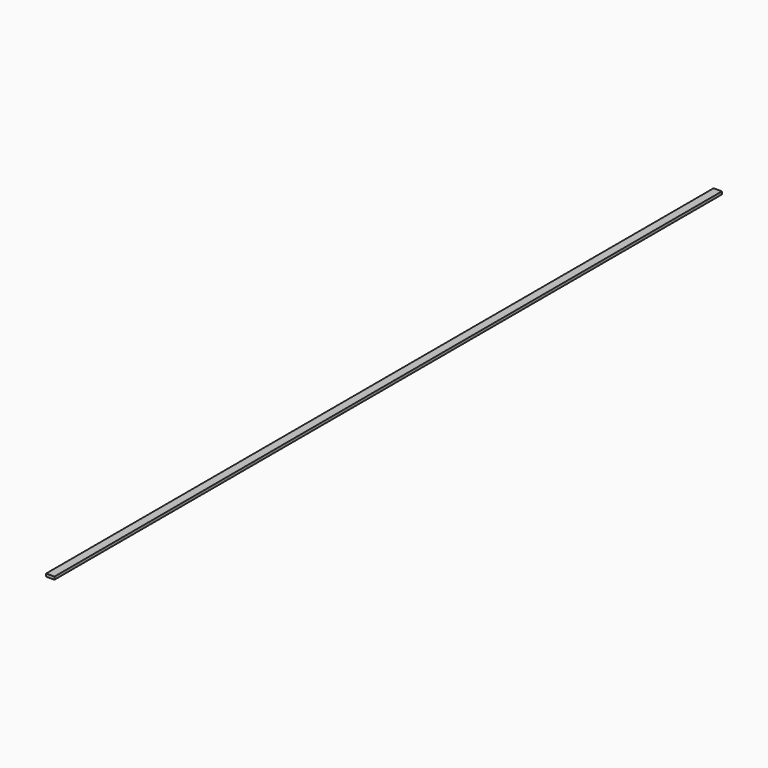
from build123d import *

# Parameters (mm, degrees)
F0_W     = 0.6
F0_H     = 60
F1_DEPTH = 0.1
F2_DEPTH = 0.1


# Not quite as in the source:
# - a feature names something its author has since deleted; it is built from what else it names


with BuildPart() as f1:
    # F0 (on Top) → F1 (new body)
    with BuildSketch(Plane.XY):
        with Locations((-0.3, -30)):
            Rectangle(F0_W, F0_H)
    extrude(amount=F1_DEPTH)

    # F2 (add): a face of the model
    f2_faces = [f1.faces().sort_by_distance(p)[0] for p in [
        (-0.3, -30, 0.1),
    ]]
    extrude(f2_faces, amount=F2_DEPTH)


solid = f1.part
